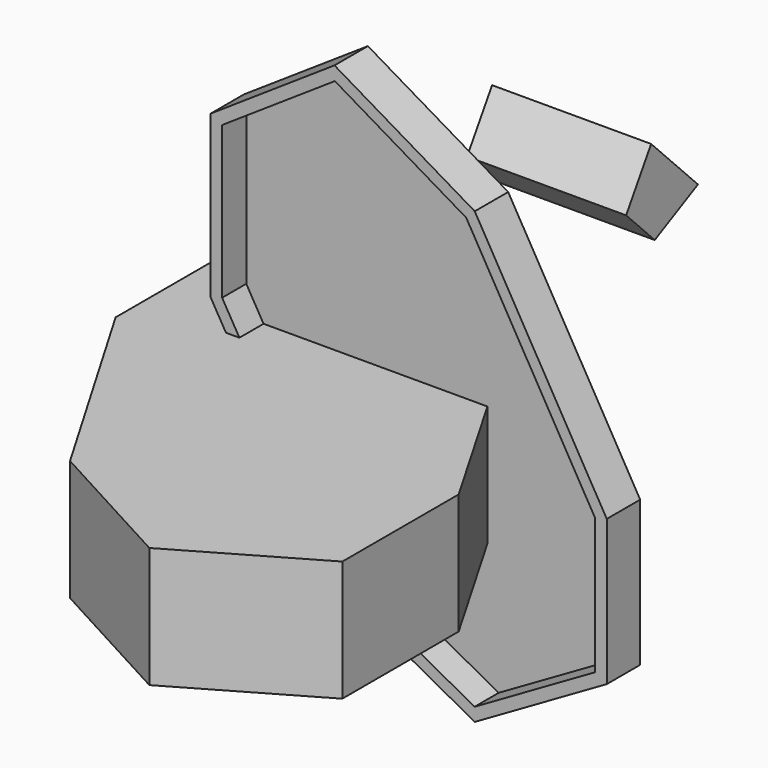
from build123d import *

# Parameters (mm, degrees)
F2_DEPTH  = 26.416
F3_T      = -2.54
F4_DEPTH  = 34.798
F5_T      = -2.54
F10_DEPTH = 9.144
F11_T     = -2.54


# Not quite as in the source:
# - a feature of the source that left no trace in its solid (it failed there, or was rolled back) is left out


with BuildPart() as f2:
    # F0 (on Top) → F2 (new body)
    with BuildSketch(Plane.XY):
        Polygon((-57.8209497035, 18.8549458981), (-57.8209497035, -16.4633058012), (-30.6930541992, -62.8396645188), (0, -79.508036375), (28.8835763931, -62.8396645188), (28.8835763931, -31.0100559145), (0, 18.8549458981), (-30.6930541992, 36.9788259268), align=None)
    extrude(amount=-F2_DEPTH)

    # F3
    f3_openings = [f2.faces().sort_by_distance(p)[0] for p in [
        (-15.016134, -21.984576, -26.416),
    ]]
    offset(amount=F3_T, openings=f3_openings)


with BuildPart() as f4:
    # F1 (on Right) → F4 (new body)
    with BuildSketch(Plane.YZ):
        Polygon((27.0421076566, 38.0343087018), (14.2326252535, 51.0408654809), (7.3943502405, 40.0662297715), (15.2179701254, 32.1222431958), align=None)
    extrude(amount=F4_DEPTH)

    # F5
    f5_openings = [f4.faces().sort_by_distance(p)[0] for p in [
        (17.399, 20.637366, 44.537587),
    ]]
    offset(amount=F5_T, openings=f5_openings)


with BuildPart() as f10:
    # F9 (on Front) → F10 (new body)
    with BuildSketch(Plane.XZ):
        Polygon((-42.9133428261, 41.1014470737), (-42.9133428261, 5.7831953745), (-15.7854473218, -40.5931633431), (14.9076068774, -57.2615351994), (43.7911832705, -40.5931633431), (43.7911832705, -8.7635547388), (14.9076068774, 41.1014470737), (-15.7854473218, 59.2253271025), align=None)
    extrude(amount=F10_DEPTH)

    # F11
    f11_openings = [f10.faces().sort_by_distance(p)[0] for p in [
        (-0.108527, -9.144, 0.261925),
    ]]
    offset(amount=F11_T, openings=f11_openings)


solid = Compound([f2.part, f4.part, f10.part])
